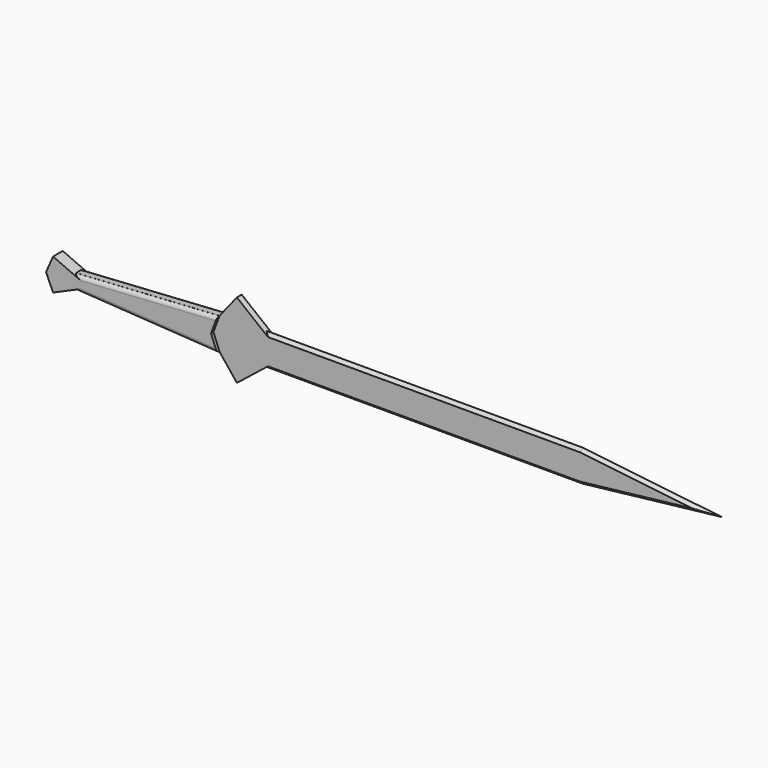
from build123d import *

# Parameters (mm, degrees)
F1_DEPTH = 1.27
F2_R     = 0.762
F3_DEPTH = 0.635
F4_SIZE  = 0.63499


# Not quite as in the source:
# - a fillet or chamfer is up to 0.001 mm smaller than in the source, because OpenCascade refuses the exact size


with BuildPart() as f1:
    # F0 (on Front) → F1 (new body, symmetric)
    with BuildSketch(Plane.XZ):
        Polygon((-30.9530049562, -3.3370526507), (-30.1719289273, -1.8979058368), (-34.4893708825, 0), (-35.9563070381, -3.3370526507), align=None)
        Polygon((-30.1719289273, -4.7761994647), (-30.9530049562, -3.3370526507), (-35.9563070381, -3.3370526507), (-34.4893708825, -6.6741053015), align=None)
        Polygon((-1.278280112, -3.4174603466), (0, 0), (-30.1719289273, -1.8979058368), (-30.9530049562, -3.3370526507), align=None)
        Polygon((0, -6.6741053015), (-1.278280112, -3.4174603466), (-30.9530049562, -3.3370526507), (-30.1719289273, -4.7761994647), align=None)
    extrude(amount=F1_DEPTH, both=True)

    # F2
    f2_edges = [f1.edges().sort_by_distance(p)[0] for p in [
        (-15.085964, -1.27, -0.948953),
        (-15.085964, 1.27, -0.948953),
        (-15.085964, 1.27, -5.725152),
        (-15.085964, -1.27, -5.725152),
    ]]
    fillet(f2_edges, radius=F2_R)

    # F0 (on Front) → F3 (join, symmetric)
    with BuildSketch(Plane.XZ):
        Polygon((-1.278280112, -3.4174603466), (0, 0), (-30.1719289273, -1.8979058368), (-30.9530049562, -3.3370526507), align=None)
        Polygon((3.6480247509, 4.5782560483), (0, 0), (-1.278280112, -3.4174603466), (105.1078885794, -3.3370526507), (75.8452340961, 0), (9.3937172488, 0), align=None)
        Polygon((-30.9530049562, -3.3370526507), (-30.1719289273, -1.8979058368), (-34.4893708825, 0), (-35.9563070381, -3.3370526507), align=None)
        Polygon((105.1078885794, -3.3370526507), (-1.278280112, -3.4174603466), (0, -6.6741053015), (3.6480247509, -11.2523613498), (9.3937172488, -6.6741053015), (75.8452340961, -6.6741053015), align=None)
        Polygon((0, -6.6741053015), (-1.278280112, -3.4174603466), (-30.9530049562, -3.3370526507), (-30.1719289273, -4.7761994647), align=None)
        Polygon((-30.1719289273, -4.7761994647), (-30.9530049562, -3.3370526507), (-35.9563070381, -3.3370526507), (-34.4893708825, -6.6741053015), align=None)
    extrude(amount=F3_DEPTH, both=True)

    # F4 (size 0.635 in the source; OpenCascade refuses exactly that, so slightly less here)
    f4_edges = [f1.edges().sort_by_distance(p)[0] for p in [
        (42.619476, -0.635, -6.674105),
        (42.619476, 0.635, -6.674105),
        (42.619476, -0.635, 0),
        (42.619476, 0.635, 0),
        (90.476561, -0.635, -1.668526),
        (90.476561, 0.635, -1.668526),
        (90.476561, -0.635, -5.005579),
        (90.476561, 0.635, -5.005579),
    ]]
    chamfer(f4_edges, length=F4_SIZE)


solid = f1.part
